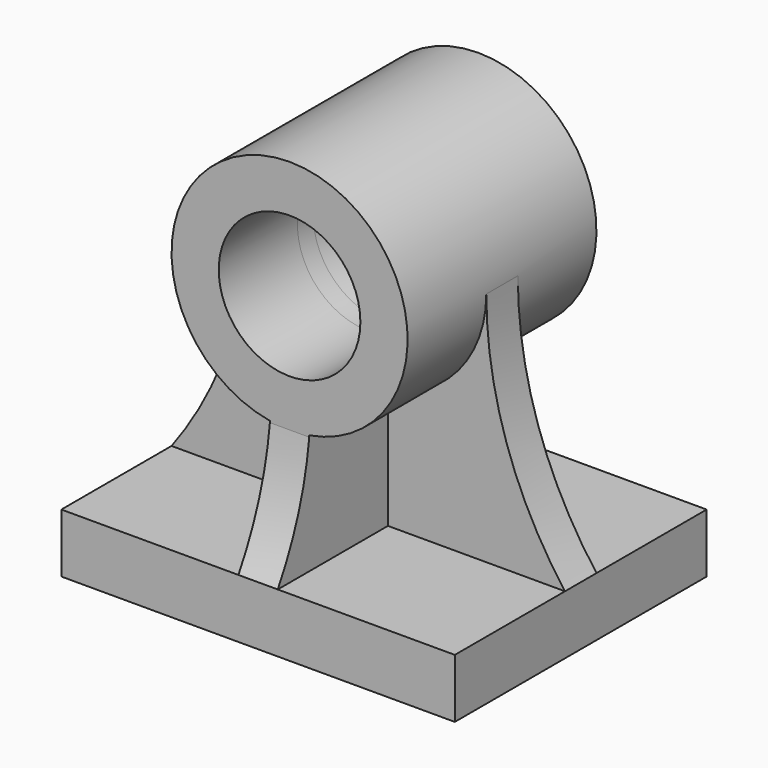
from build123d import *
from build123d import SkipClean  # not in build123d's __all__

# Parameters (mm, degrees)
F0_W     = 100
F0_H     = 15
F1_DEPTH = 40
F0_R     = 18
F2_DEPTH = 5
F3_DEPTH = 30
F5_DEPTH = 5


# Not quite as in the source:
# - a pattern or mirror of a feature is missing from the dataset's text; its kind, count and spacing are read off the source's solid


with BuildPart() as f1:
    # F0 (on Front) → F1 (new body, symmetric)
    with BuildSketch(Plane.XZ):
        with Locations((0, 7.5)):
            Rectangle(F0_W, F0_H)
    extrude(amount=F1_DEPTH, both=True)

    # F0 (on Front) → F2 (join, symmetric)
    with BuildSketch(Plane.XZ):
        with BuildLine():
            ThreePointArc((-30, 75), (-35.1316701949, 43.3772233983), (-50, 15))
            Line((-50, 15), (50, 15))
            ThreePointArc((50, 15), (35.1316701949, 43.3772233983), (30, 75))
            ThreePointArc((30, 75), (0, 45), (-30, 75))
        make_face()
        with Locations((0, 7.5)):
            Rectangle(F0_W, F0_H)
        with BuildLine():
            ThreePointArc((30, 75), (0, 105), (-30, 75))
            ThreePointArc((-30, 75), (0, 45), (30, 75))
        make_face()
        with Locations((0, 75)):
            Circle(F0_R, mode=Mode.SUBTRACT)
    extrude(amount=F2_DEPTH, both=True)

    # F0 (on Front) → F3 (join, symmetric)
    with BuildSketch(Plane.XZ):
        with BuildLine():
            ThreePointArc((30, 75), (0, 105), (-30, 75))
            ThreePointArc((-30, 75), (0, 45), (30, 75))
        make_face()
        with Locations((0, 75)):
            Circle(F0_R, mode=Mode.SUBTRACT)
    with SkipClean():  # cleaning this boolean's faces spoils the solid; the shape is the same uncleaned
        extrude(amount=F3_DEPTH, both=True)

    # F4 (on Right) → F5 (join, symmetric)
    with BuildSketch(Plane.YZ):
        with BuildLine():
            ThreePointArc((40, 15), (33.4008913624, 29.4669637875), (30, 45))
            Line((30, 45), (30, 50))
            Line((30, 50), (5, 50))
            Line((5, 50), (5, 15))
            Line((5, 15), (40, 15))
        make_face()
    f5 = extrude(amount=F5_DEPTH, both=True)

    # F5_copies: F5 across plane
    add(f5.mirror(Plane(origin=(0, 0, 0), x_dir=(0, 0, -1), z_dir=(0, -1, 0))), clean=False)


solid = f1.part
